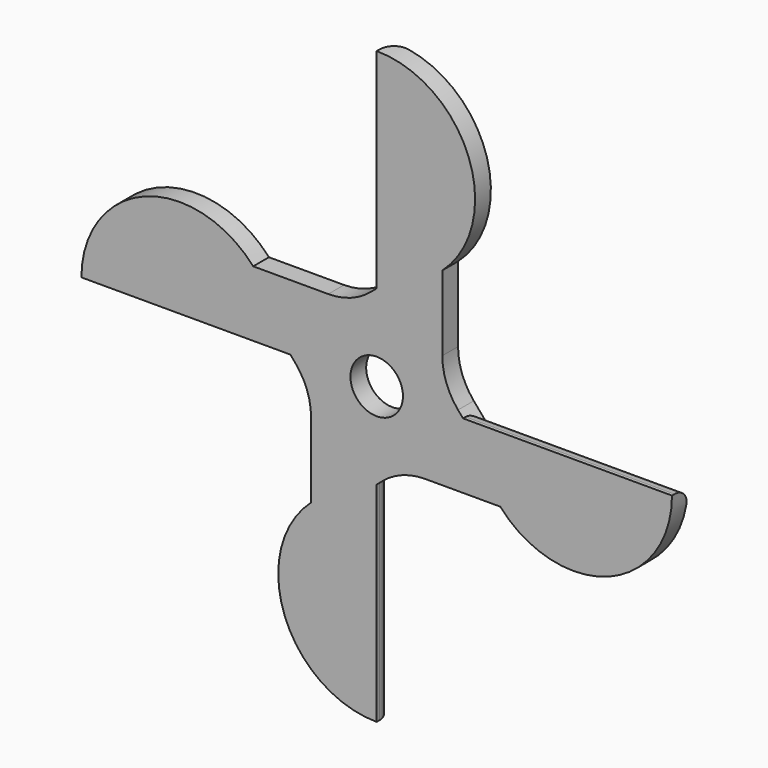
from build123d import *

# Parameters (mm, degrees)
F0_R     = 3.75
F1_DEPTH = 5
F3_DEPTH = 3
F4_R     = 55.5278104075
F5_DEPTH = 5
F6_R     = 2.5
F7_R     = 4
F8_DEPTH = 3.0010001


with BuildPart() as f1:
    # F0 (on Front) → F1 (new body)
    with BuildSketch(Plane.XZ):
        with BuildLine():
            Line((10, 7.379066267), (10, 18.8196601125))
            ThreePointArc((10, 18.8196601125), (14.0125853844, 35.3523313466), (0, 45))
            Line((0, 45), (0, 43))
            ThreePointArc((0, 43), (11.7683072321, 35.5233092337), (10, 21.6933761371))
            Line((10, 21.6933761371), (0, 13.1515390832))
            Line((0, 13.1515390832), (-0.8841328604, 12.3963272004))
            ThreePointArc((-0.8841328604, 12.3963272004), (-3.9176162816, 10.618189727), (-7.379066267, 10))
            Line((-7.379066267, 10), (-18.8196601125, 10))
            ThreePointArc((-18.8196601125, 10), (-35.3523313466, 14.0125853844), (-45, 0))
            Line((-45, 0), (-43, 0))
            ThreePointArc((-43, 0), (-35.5233092337, 11.7683072321), (-21.6933761371, 10))
            Line((-21.6933761371, 10), (-12.3963272004, -0.8841328604))
            ThreePointArc((-12.3963272004, -0.8841328604), (-10.618189727, -3.9176162816), (-10, -7.379066267))
            Line((-10, -7.379066267), (-10, -18.8196601125))
            ThreePointArc((-10, -18.8196601125), (-14.0125853844, -35.3523313466), (0, -45))
            Line((0, -45), (0, -43))
            ThreePointArc((0, -43), (-11.7683072321, -35.5233092337), (-10, -21.6933761371))
            Line((-10, -21.6933761371), (0.8841328604, -12.3963272004))
            ThreePointArc((0.8841328604, -12.3963272004), (3.9176162816, -10.618189727), (7.379066267, -10))
            Line((7.379066267, -10), (18.8196601125, -10))
            ThreePointArc((18.8196601125, -10), (35.3523313466, -14.0125853844), (45, 0))
            Line((45, 0), (43, 0))
            ThreePointArc((43, 0), (35.5233092337, -11.7683072321), (21.6933761371, -10))
            Line((21.6933761371, -10), (12.3963272004, 0.8841328604))
            ThreePointArc((12.3963272004, 0.8841328604), (10.618189727, 3.9176162816), (10, 7.379066267))
        make_face()
        Circle(F0_R, mode=Mode.SUBTRACT)
    extrude(amount=F1_DEPTH)

    # F2 (on face) → F3 (join)
    with BuildSketch(Plane(origin=(0, 0, 0), x_dir=(-1, 0, 0), z_dir=(0, 1, 0))):
        with BuildLine():
            Line((0, 43), (0, 45))
            ThreePointArc((0, 45), (-14.0125853844, 35.3523313466), (-10, 18.8196601125))
            Line((-10, 18.8196601125), (-10, 7.379066267))
            ThreePointArc((-10, 7.379066267), (-10.618189727, 3.9176162816), (-12.3963272004, 0.8841328604))
            Line((-12.3963272004, 0.8841328604), (-13.1515390832, 0))
            Line((-13.1515390832, 0), (-9.8753882025, 0))
            Line((-9.8753882025, 0), (-3.75, 0))
            ThreePointArc((-3.75, 0), (-2.6516504294, 2.6516504294), (0, 3.75))
            Line((0, 3.75), (0, 9.8753882025))
            Line((0, 9.8753882025), (0, 13.1515390832))
            Line((0, 13.1515390832), (-10, 21.6933761371))
            ThreePointArc((-10, 21.6933761371), (-11.7683072321, 35.5233092337), (0, 43))
        make_face()
        with BuildLine():
            Line((0, 13.1515390832), (0, 43))
            ThreePointArc((0, 43), (-11.7683072321, 35.5233092337), (-10, 21.6933761371))
            Line((-10, 21.6933761371), (0, 13.1515390832))
        make_face()
        with BuildLine():
            Line((0.8841328604, 12.3963272004), (0, 13.1515390832))
            Line((0, 13.1515390832), (0, 9.8753882025))
            Line((0, 9.8753882025), (0, 3.75))
            ThreePointArc((0, 3.75), (2.6516504294, 2.6516504294), (3.75, 0))
            Line((3.75, 0), (9.8753882025, 0))
            Line((9.8753882025, 0), (13.1515390832, 0))
            Line((13.1515390832, 0), (21.6933761371, 10))
            ThreePointArc((21.6933761371, 10), (35.5233092337, 11.7683072321), (43, 0))
            Line((43, 0), (45, 0))
            ThreePointArc((45, 0), (35.3523313466, 14.0125853844), (18.8196601125, 10))
            Line((18.8196601125, 10), (7.379066267, 10))
            ThreePointArc((7.379066267, 10), (3.9176162816, 10.618189727), (0.8841328604, 12.3963272004))
        make_face()
        with BuildLine():
            Line((-21.6933761371, -10), (-13.1515390832, 0))
            Line((-13.1515390832, 0), (-43, 0))
            ThreePointArc((-43, 0), (-35.5233092337, -11.7683072321), (-21.6933761371, -10))
        make_face()
        with BuildLine():
            Line((-9.8753882025, 0), (-13.1515390832, 0))
            Line((-13.1515390832, 0), (-21.6933761371, -10))
            ThreePointArc((-21.6933761371, -10), (-35.5233092337, -11.7683072321), (-43, 0))
            Line((-43, 0), (-45, 0))
            ThreePointArc((-45, 0), (-35.3523313466, -14.0125853844), (-18.8196601125, -10))
            Line((-18.8196601125, -10), (-7.379066267, -10))
            ThreePointArc((-7.379066267, -10), (-3.9176162816, -10.618189727), (-0.8841328604, -12.3963272004))
            Line((-0.8841328604, -12.3963272004), (0, -13.1515390832))
            Line((0, -13.1515390832), (0, -9.8753882025))
            Line((0, -9.8753882025), (0, -3.75))
            ThreePointArc((0, -3.75), (-2.6516504294, -2.6516504294), (-3.75, 0))
            Line((-3.75, 0), (-9.8753882025, 0))
        make_face()
        with BuildLine():
            ThreePointArc((3.75, 0), (2.6516504294, 2.6516504294), (0, 3.75))
            ThreePointArc((0, 3.75), (-2.6516504294, 2.6516504294), (-3.75, 0))
            ThreePointArc((-3.75, 0), (-2.6516504294, -2.6516504294), (0, -3.75))
            ThreePointArc((0, -3.75), (2.6516504294, -2.6516504294), (3.75, 0))
        make_face()
        with BuildLine():
            Line((9.8753882025, 0), (3.75, 0))
            ThreePointArc((3.75, 0), (2.6516504294, -2.6516504294), (0, -3.75))
            Line((0, -3.75), (0, -9.8753882025))
            Line((0, -9.8753882025), (0, -13.1515390832))
            Line((0, -13.1515390832), (10, -21.6933761371))
            ThreePointArc((10, -21.6933761371), (11.7683072321, -35.5233092337), (0, -43))
            Line((0, -43), (0, -45))
            ThreePointArc((0, -45), (14.0125853844, -35.3523313466), (10, -18.8196601125))
            Line((10, -18.8196601125), (10, -7.379066267))
            ThreePointArc((10, -7.379066267), (10.618189727, -3.9176162816), (12.3963272004, -0.8841328604))
            Line((12.3963272004, -0.8841328604), (13.1515390832, 0))
            Line((13.1515390832, 0), (9.8753882025, 0))
        make_face()
        with BuildLine():
            Line((21.6933761371, 10), (13.1515390832, 0))
            Line((13.1515390832, 0), (43, 0))
            ThreePointArc((43, 0), (35.5233092337, 11.7683072321), (21.6933761371, 10))
        make_face()
        with BuildLine():
            Line((10, -21.6933761371), (0, -13.1515390832))
            Line((0, -13.1515390832), (0, -43))
            ThreePointArc((0, -43), (11.7683072321, -35.5233092337), (10, -21.6933761371))
        make_face()
    extrude(amount=F3_DEPTH)

    # F4 (on face) → F5 (cut)
    with BuildSketch(Plane.XZ.offset(5)):
        Circle(F4_R)
    extrude(amount=-F5_DEPTH, mode=Mode.SUBTRACT)

    # F6
    f6_edges = [f1.edges().sort_by_distance(p)[0] for p in [
        (29.07577, 3, 0),
        (0, 3, 29.07577),
        (-29.07577, 3, 0),
        (0, 3, -29.07577),
    ]]
    fillet(f6_edges, radius=F6_R)

    # F7 (on face) → F8 (cut, through all)
    with BuildSketch(Plane.XZ):
        Circle(F7_R)
    extrude(amount=-F8_DEPTH, mode=Mode.SUBTRACT)


solid = f1.part
